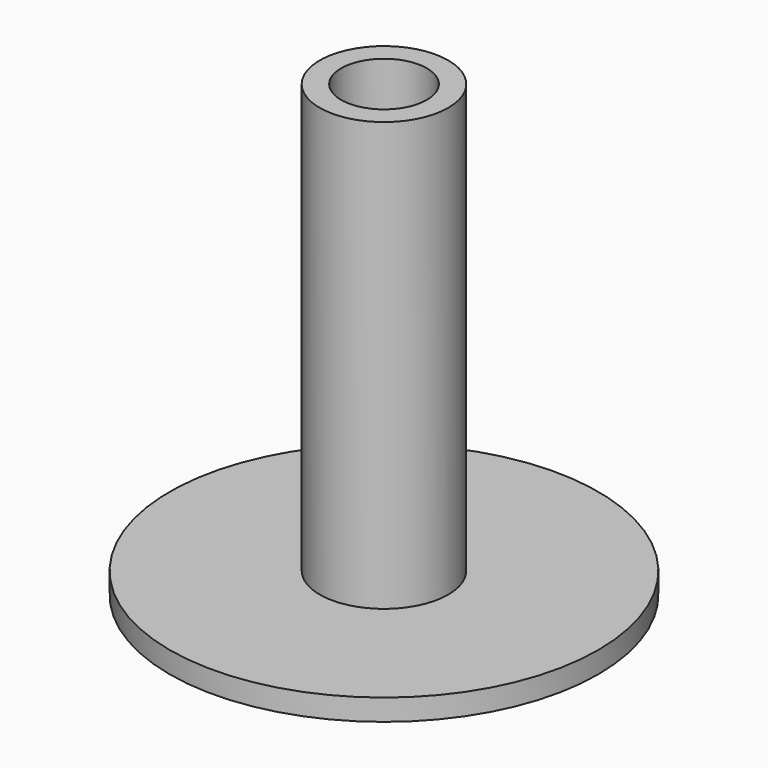
from build123d import *

# Parameters (mm, degrees)
F0_R            = 63.5
F1_DEPTH        = 6.35
F2_R            = 0.7874
F3_DEPTH        = 3.175
F3_COPIES_COUNT = 4
F4_R            = 19.05
F5_DEPTH        = 6.35
F6_R            = 19.05
F7_DEPTH        = 127
F8_R            = 12.7
F9_DEPTH        = 139.701


# Not quite as in the source:
# - a pattern or mirror of a feature is missing from the dataset's text; its kind, count and spacing are read off the source's solid


with BuildPart() as f1:
    # F0 (on Top) → F1 (new body)
    with BuildSketch(Plane.XY):
        Circle(F0_R)
    extrude(amount=F1_DEPTH)

    # F2 (on face) → F3 (join)
    with BuildSketch(Plane(origin=(0, 0, 0), x_dir=(1, 0, 0), z_dir=(0, 0, -1))):
        with Locations((-30.1625, 0)):
            Circle(F2_R)
    f3 = extrude(amount=F3_DEPTH)

    # F3_copies: F3 ×4 about axis
    f3_copies_axis = Axis((0, 0, 0), (0, 0, 1))
    for i in range(1, F3_COPIES_COUNT):
        add(f3.rotate(f3_copies_axis, i * 360 / F3_COPIES_COUNT))

    # F4 (on face) → F5 (join)
    with BuildSketch(Plane(origin=(0, 0, 0), x_dir=(1, 0, 0), z_dir=(0, 0, -1))):
        Circle(F4_R)
    extrude(amount=F5_DEPTH)

    # F6 (on face) → F7 (join)
    with BuildSketch(Plane.XY.offset(6.35)):
        Circle(F6_R)
    extrude(amount=F7_DEPTH)

    # F8 (on face) → F9 (cut, through all)
    with BuildSketch(Plane.XY.offset(133.35)):
        Circle(F8_R)
    extrude(amount=-F9_DEPTH, mode=Mode.SUBTRACT)


solid = f1.part
